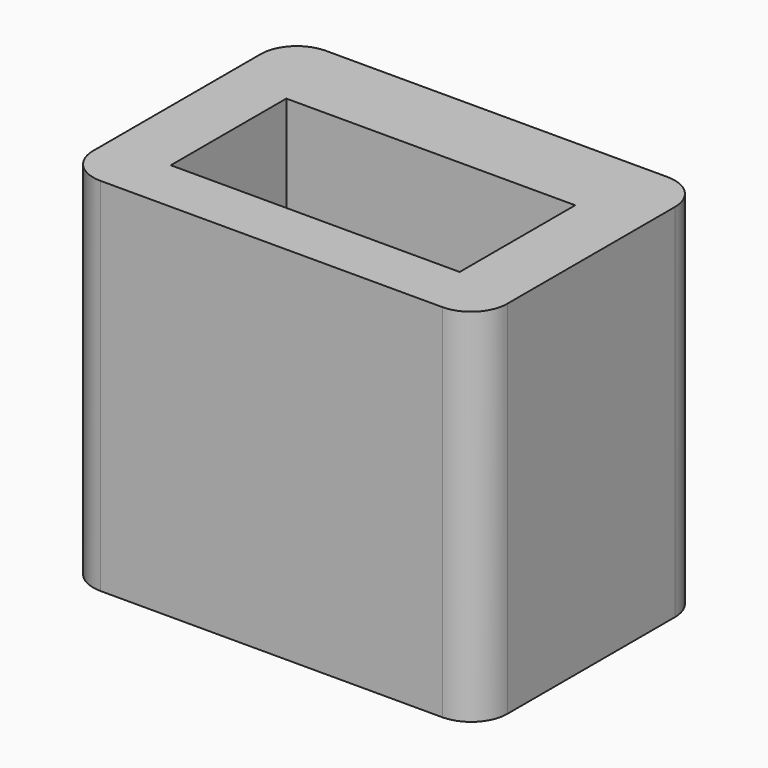
from build123d import *

# Parameters (mm, degrees)
F0_W     = 17.2
F0_H     = 11.7
F0_W_2   = 12
F0_H_2   = 6
F1_DEPTH = 15
F2_R     = 1.5
F0_R     = 2.25
F3_DEPTH = 1.5


# Not quite as in the source:
# - a feature names something its author has since deleted; it is built from what else it names


with BuildPart() as f1:
    # F0 (on Top) → F1 (new body)
    with BuildSketch(Plane.XY):
        with Locations((0, 0.571324781)):
            Rectangle(F0_W, F0_H)
        Rectangle(F0_W_2, F0_H_2, mode=Mode.SUBTRACT)
    extrude(amount=F1_DEPTH)

    # F2
    f2_edges = [f1.edges().sort_by_distance(p)[0] for p in [
        (-8.6, 6.421325, 7.5),
        (8.6, 6.421325, 7.5),
        (8.6, -5.278675, 7.5),
        (-8.6, -5.278675, 7.5),
    ]]
    fillet(f2_edges, radius=F2_R)

    # F0 (on Top) → F3 (join)
    with BuildSketch(Plane.XY):
        Rectangle(F0_W_2, F0_H_2)
        Circle(F0_R, mode=Mode.SUBTRACT)
    extrude(amount=F3_DEPTH)


solid = f1.part
